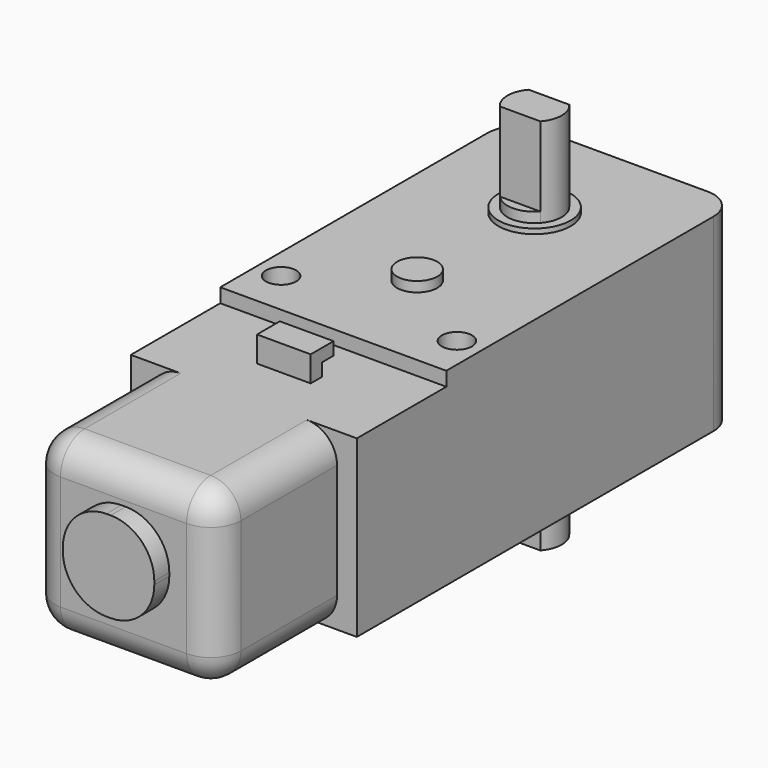
from build123d import *

# Parameters (mm, degrees)
F0_R      = 1.5
F0_R_2    = 3.6
F1_DEPTH  = 9.4
F0_W      = 5
F0_H      = 5
F0_R_3    = 0.7
F2_DEPTH  = 1.3
F0_W_2    = 5.3451308049
F0_H_2    = 2.8401017189
F3_DEPTH  = 9.4
F4_DEPTH  = 8
F0_W_3    = 9.1007668525
F0_H_3    = 1.8676674664
F5_DEPTH  = 4.5
F6_R      = 3
F7_R      = 4.3340927557
F9_DEPTH  = 5.3451308049
F10_R     = 2
F11_DEPTH = 1
F10_R_2   = 3.6
F10_R_3   = 2.7
F12_DEPTH = 0.5
F13_DEPTH = 18.8
F14_DEPTH = 10.9


with BuildPart() as f1:
    # F0 (on Top) → F1 (new body, symmetric)
    with BuildSketch(Plane.XY):
        with BuildLine():
            Line((-11.25, 8.2), (-11.25, -25.0427096879))
            Line((-11.25, -25.0427096879), (11.25, -25.0427096879))
            Line((11.25, -25.0427096879), (11.25, 8.2))
            ThreePointArc((11.25, 8.2), (10.3713203436, 10.3213203436), (8.25, 11.2))
            Line((8.25, 11.2), (2.5, 11.2))
            Line((2.5, 11.2), (-2.5, 11.2))
            Line((-2.5, 11.2), (-8.25, 11.2))
            ThreePointArc((-8.25, 11.2), (-10.3713203436, 10.3213203436), (-11.25, 8.2))
        make_face()
        with Locations((-8.75, -20.6)):
            Circle(F0_R, mode=Mode.SUBTRACT)
        with Locations((8.75, -20.6)):
            Circle(F0_R, mode=Mode.SUBTRACT)
        Circle(F0_R_2, mode=Mode.SUBTRACT)
        Circle(F0_R_2)
        with BuildLine():
            ThreePointArc((2.0124611797, 1.8), (2.5222653692, 0.9634196424), (2.7, 0))
            ThreePointArc((2.7, 0), (2.5222653692, -0.9634196424), (2.0124611797, -1.8))
            ThreePointArc((2.0124611797, -1.8), (0, -2.7), (-2.0124611797, -1.8))
            ThreePointArc((-2.0124611797, -1.8), (-2.7, 0), (-2.0124611797, 1.8))
            ThreePointArc((-2.0124611797, 1.8), (0, 2.7), (2.0124611797, 1.8))
        make_face(mode=Mode.SUBTRACT)
    extrude(amount=F1_DEPTH, both=True)

    # F0 (on Top) → F2 (join, symmetric)
    with BuildSketch(Plane.XY):
        with Locations((0, 13.7)):
            Rectangle(F0_W, F0_H)
        with Locations((0, 13.6)):
            Circle(F0_R_3, mode=Mode.SUBTRACT)
    extrude(amount=F2_DEPTH, both=True)

    # F0 (on Top) → F3 (join)
    with BuildSketch(Plane.XY):
        Polygon((11.25, -25.0427096879), (-11.25, -25.0427096879), (-11.25, -36.1717492342), (-9.2768007889, -36.1717492342), (9.2768007889, -36.1717492342), (11.25, -36.1717492342), align=None)
        with Locations((0, -29.7719910741)):
            Rectangle(F0_W_2, F0_H_2, mode=Mode.SUBTRACT)
        with BuildLine():
            Line((9.2768007889, -36.1717492342), (-9.2768007889, -36.1717492342))
            Line((-9.2768007889, -36.1717492342), (-9.2768007889, -48.1323325336))
            ThreePointArc((-9.2768007889, -48.1323325336), (-8.3981211325, -50.2536528772), (-6.2768007889, -51.1323325336))
            Line((-6.2768007889, -51.1323325336), (-4.5503834262, -51.1323325336))
            Line((-4.5503834262, -51.1323325336), (4.5503834262, -51.1323325336))
            Line((4.5503834262, -51.1323325336), (6.2768007889, -51.1323325336))
            ThreePointArc((6.2768007889, -51.1323325336), (8.3981211325, -50.2536528772), (9.2768007889, -48.1323325336))
            Line((9.2768007889, -48.1323325336), (9.2768007889, -36.1717492342))
        make_face()
        with Locations((0, -29.7719910741)):
            Rectangle(F0_W_2, F0_H_2)
    extrude(amount=-F3_DEPTH)

    # F0 (on Top) → F4 (join)
    with BuildSketch(Plane.XY):
        Polygon((11.25, -25.0427096879), (-11.25, -25.0427096879), (-11.25, -36.1717492342), (-9.2768007889, -36.1717492342), (9.2768007889, -36.1717492342), (11.25, -36.1717492342), align=None)
        with Locations((0, -29.7719910741)):
            Rectangle(F0_W_2, F0_H_2, mode=Mode.SUBTRACT)
        with BuildLine():
            Line((9.2768007889, -36.1717492342), (-9.2768007889, -36.1717492342))
            Line((-9.2768007889, -36.1717492342), (-9.2768007889, -48.1323325336))
            ThreePointArc((-9.2768007889, -48.1323325336), (-8.3981211325, -50.2536528772), (-6.2768007889, -51.1323325336))
            Line((-6.2768007889, -51.1323325336), (-4.5503834262, -51.1323325336))
            Line((-4.5503834262, -51.1323325336), (4.5503834262, -51.1323325336))
            Line((4.5503834262, -51.1323325336), (6.2768007889, -51.1323325336))
            ThreePointArc((6.2768007889, -51.1323325336), (8.3981211325, -50.2536528772), (9.2768007889, -48.1323325336))
            Line((9.2768007889, -48.1323325336), (9.2768007889, -36.1717492342))
        make_face()
    extrude(amount=F4_DEPTH)

    # F0 (on Top) → F5 (join, symmetric)
    with BuildSketch(Plane.XY):
        with Locations((0, -52.0661662668)):
            Rectangle(F0_W_3, F0_H_3)
    extrude(amount=F5_DEPTH, both=True)

    # F6
    f6_edges = [f1.edges().sort_by_distance(p)[0] for p in [
        (0, -51.132333, -9.4),
        (0, -51.132333, 8),
        (-9.276801, -42.152041, -9.4),
        (-8.398121, -50.253653, -9.4),
        (8.398121, -50.253653, -9.4),
        (9.276801, -42.152041, -9.4),
        (-9.276801, -42.152041, 8),
        (-8.398121, -50.253653, 8),
        (8.398121, -50.253653, 8),
        (9.276801, -42.152041, 8),
    ]]
    fillet(f6_edges, radius=F6_R)

    # F7
    f7_edges = [f1.edges().sort_by_distance(p)[0] for p in [
        (4.550383, -52.066166, -4.5),
        (4.550383, -52.066166, 4.5),
        (-4.550383, -52.066166, -4.5),
        (-4.550383, -52.066166, 4.5),
    ]]
    fillet(f7_edges, radius=F7_R)

    # F8 (on face) → F9 (join, through all)
    with BuildSketch(Plane.YZ.offset(-2.6725654025)):
        Polygon((-31.1920419335, 10.55), (-31.1920419335, 8), (-29.7719910741, 8), (-29.7719910741, 9.275), (-28.3519402146, 9.275), (-28.3519402146, 10.55), align=None)
        Polygon((-29.7719910741, 8), (-31.1920419335, 8), (-31.1920419335, 0), (-28.3519402146, 0), (-28.3519402146, 8), align=None)
        Polygon((-28.3519402146, 0), (-31.1920419335, 0), (-31.1920419335, -9.4), (-31.1920419335, -11.95), (-28.3519402146, -11.95), (-28.3519402146, -10.675), (-29.7719910741, -10.675), (-29.7719910741, -9.4), (-28.3519402146, -9.4), align=None)
    extrude(amount=F9_DEPTH)

    # F10 (on face) → F11 (join)
    with BuildSketch(Plane.XY.offset(9.4)):
        with Locations((0, -14.6034881473)):
            Circle(F10_R)
    extrude(amount=F11_DEPTH)

    # F10 (on face) → F12 (join)
    with BuildSketch(Plane.XY.offset(9.4)):
        Circle(F10_R_2)
        Circle(F10_R_3, mode=Mode.SUBTRACT)
    extrude(amount=F12_DEPTH)


with BuildPart() as f13:
    # F0 (on Top) → F13 (new body, symmetric)
    with BuildSketch(Plane.XY):
        with BuildLine():
            ThreePointArc((2.0124611797, -1.8), (2.5222653692, -0.9634196424), (2.7, 0))
            ThreePointArc((2.7, 0), (2.5222653692, 0.9634196424), (2.0124611797, 1.8))
            Line((2.0124611797, 1.8), (-2.0124611797, 1.8))
            ThreePointArc((-2.0124611797, 1.8), (-2.7, 0), (-2.0124611797, -1.8))
            Line((-2.0124611797, -1.8), (2.0124611797, -1.8))
        make_face()
    extrude(amount=F13_DEPTH, both=True)

    # F0 (on Top) → F14 (join, symmetric)
    with BuildSketch(Plane.XY):
        with BuildLine():
            Line((-2.0124611797, 1.8), (2.0124611797, 1.8))
            ThreePointArc((2.0124611797, 1.8), (0, 2.7), (-2.0124611797, 1.8))
        make_face()
        with BuildLine():
            ThreePointArc((-2.0124611797, -1.8), (0, -2.7), (2.0124611797, -1.8))
            Line((2.0124611797, -1.8), (-2.0124611797, -1.8))
        make_face()
    extrude(amount=F14_DEPTH, both=True)


solid = Compound([f1.part, f13.part])
